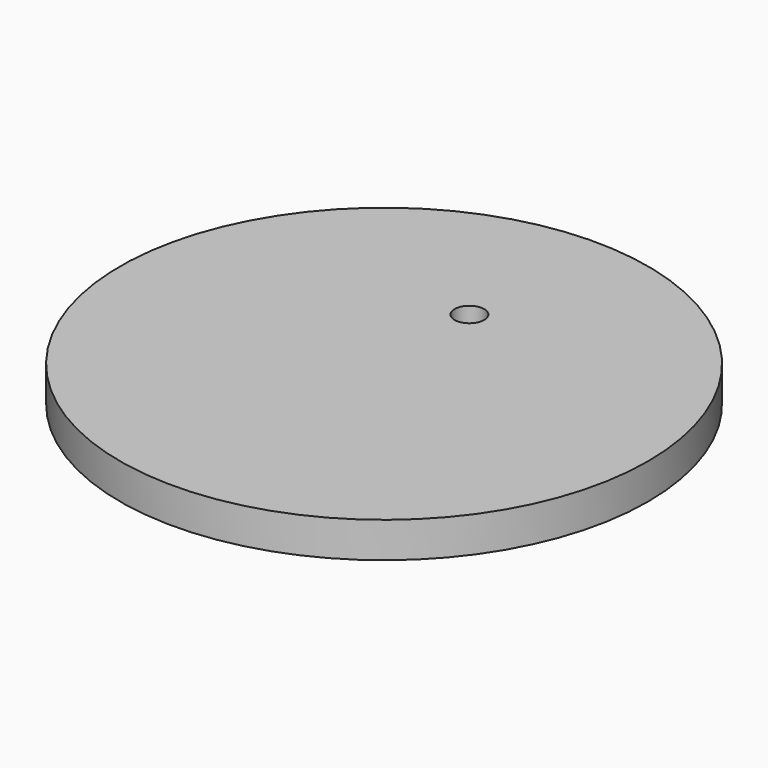
from build123d import *

# Parameters (mm, degrees)
F0_R     = 148.5
F0_R_2   = 8.3312
F1_DEPTH = 20
F2_R     = 146.5
F2_R_2   = 142
F3_DEPTH = 5


# Not quite as in the source:
# - a feature names something its author has since deleted; it is built from what else it names


with BuildPart() as f1:
    # F0 (on Top) → F1 (new body)
    with BuildSketch(Plane.XY):
        Circle(F0_R)
        with Locations((0, 60)):
            Circle(F0_R_2, mode=Mode.SUBTRACT)
    extrude(amount=F1_DEPTH)

    # F2 (on face) → F3 (cut)
    with BuildSketch(Plane.XY):
        Circle(F2_R)
        Circle(F2_R_2, mode=Mode.SUBTRACT)
    extrude(amount=F3_DEPTH, mode=Mode.SUBTRACT)


solid = f1.part
